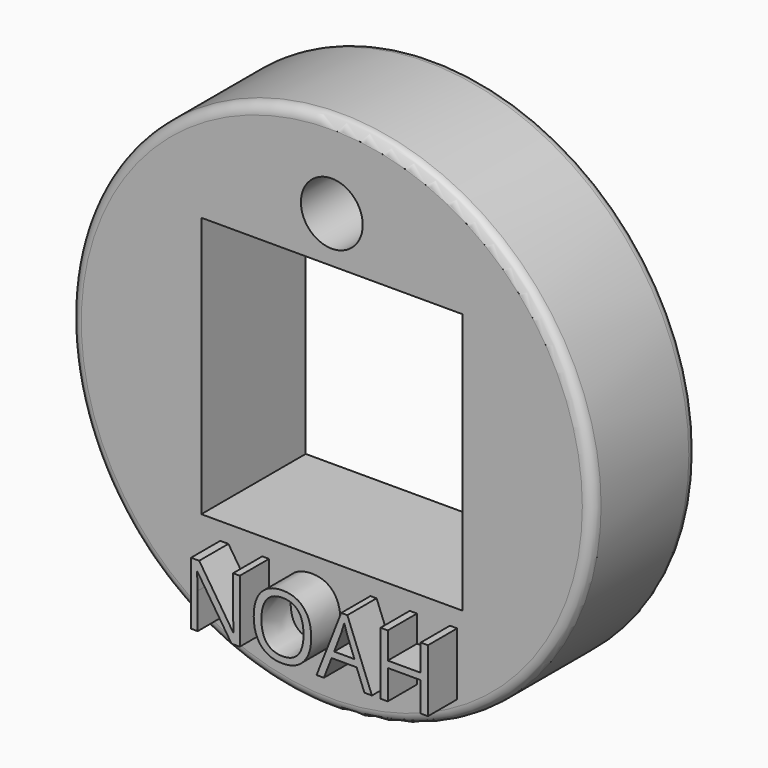
from build123d import *

# Parameters (mm, degrees)
F0_R         = 50
F1_DEPTH     = 25
F2_W         = 50
F2_H         = 50
F3_DEPTH     = 25
F4_TEXT_SIZE = 16.7669314477
F5_DEPTH     = 7
F6_R         = 2
F7_R         = 5.9223994119
F8_DEPTH     = 26


# Not quite as in the source:
# - Text() gives the source's letters only with a copy of the font that has no kerning and outlines rounded to 1/6400 em; it was checked with that copy


with BuildPart() as f1:
    # F0 (on Front) → F1 (new body)
    with BuildSketch(Plane.XZ):
        Circle(F0_R)
    extrude(amount=-F1_DEPTH)

    # F2 (on Front) → F3 (cut)
    with BuildSketch(Plane.XZ):
        Rectangle(F2_W, F2_H)
    extrude(amount=-F3_DEPTH, mode=Mode.SUBTRACT)

    # F4 (on Front) → F5 (join)
    with BuildSketch(Plane.XZ):
        with Locations((-23.0213906616, -40.2874313295)):
            Text('NOAH', F4_TEXT_SIZE, font='Open Sans', text_align=(TextAlign.LEFT, TextAlign.BOTTOM))
    extrude(amount=F5_DEPTH)

    # F6
    f6_edges = [f1.edges().sort_by_distance(p)[0] for p in [
        (-50, 0, 0),
        (-50, 25, 0),
    ]]
    fillet(f6_edges, radius=F6_R)

    # F7 (on face) → F8 (cut)
    with BuildSketch(Plane.XZ):
        with Locations((0, 33.8302142918)):
            Circle(F7_R)
    extrude(amount=-F8_DEPTH, mode=Mode.SUBTRACT)


solid = f1.part
